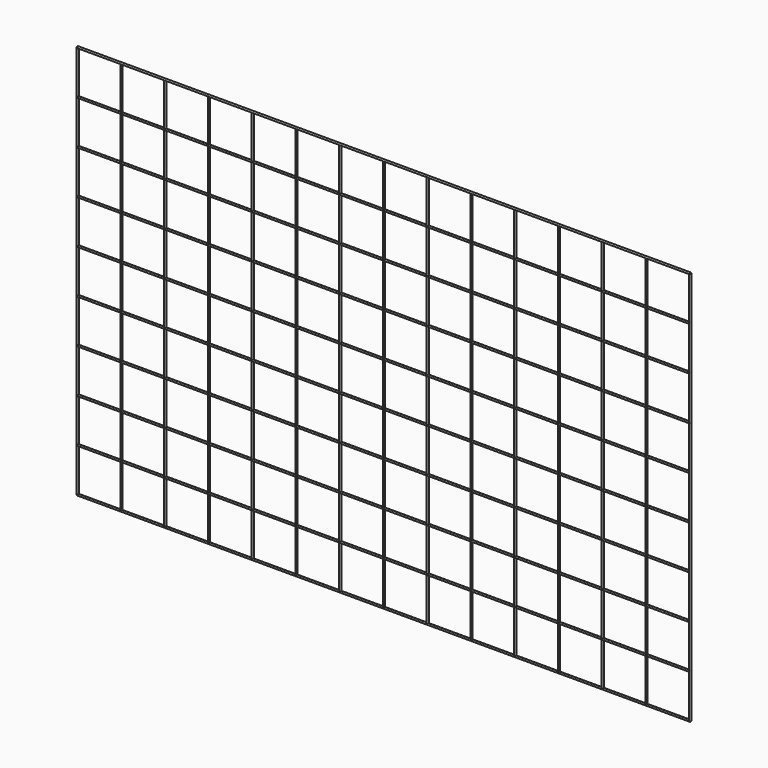
from build123d import *

# Parameters (mm, degrees)
F1_DEPTH = 2800
F2_R     = 4
F3_DEPTH = 1800


with BuildPart() as f1:
    # F0 (on Right) → F1 (new body)
    with BuildSketch(Plane.YZ):
        with BuildLine():
            ThreePointArc((4, -1800), (2.8284271247, -1797.1715728753), (0, -1796))
            ThreePointArc((0, -1796), (-2.8284271247, -1802.8284271247), (4, -1800))
        make_face()
    extrude(amount=F1_DEPTH)


with BuildPart() as f1b:
    # F0 (on Right) → F1, piece 2 (new body)
    with BuildSketch(Plane.YZ):
        with BuildLine():
            ThreePointArc((4, -1600), (2.8284271247, -1597.1715728753), (0, -1596))
            Line((0, -1596), (0, -1600))
            Line((0, -1600), (0, -1604))
            ThreePointArc((0, -1604), (2.8284271247, -1602.8284271247), (4, -1600))
        make_face()
        with BuildLine():
            Line((0, -1600), (0, -1596))
            ThreePointArc((0, -1596), (-4, -1600), (0, -1604))
            Line((0, -1604), (0, -1600))
        make_face()
    extrude(amount=F1_DEPTH)


with BuildPart() as f1c:
    # F0 (on Right) → F1, piece 3 (new body)
    with BuildSketch(Plane.YZ):
        with BuildLine():
            ThreePointArc((4, -1400), (2.8284271247, -1397.1715728753), (0, -1396))
            Line((0, -1396), (0, -1400))
            Line((0, -1400), (0, -1404))
            ThreePointArc((0, -1404), (2.8284271247, -1402.8284271247), (4, -1400))
        make_face()
        with BuildLine():
            Line((0, -1400), (0, -1396))
            ThreePointArc((0, -1396), (-4, -1400), (0, -1404))
            Line((0, -1404), (0, -1400))
        make_face()
    extrude(amount=F1_DEPTH)


with BuildPart() as f1d:
    # F0 (on Right) → F1, piece 4 (new body)
    with BuildSketch(Plane.YZ):
        with BuildLine():
            ThreePointArc((4, -1200), (2.8284271247, -1197.1715728753), (0, -1196))
            Line((0, -1196), (0, -1200))
            Line((0, -1200), (0, -1204))
            ThreePointArc((0, -1204), (2.8284271247, -1202.8284271247), (4, -1200))
        make_face()
        with BuildLine():
            Line((0, -1200), (0, -1196))
            ThreePointArc((0, -1196), (-4, -1200), (0, -1204))
            Line((0, -1204), (0, -1200))
        make_face()
    extrude(amount=F1_DEPTH)


with BuildPart() as f1e:
    # F0 (on Right) → F1, piece 5 (new body)
    with BuildSketch(Plane.YZ):
        with BuildLine():
            ThreePointArc((4, -1000), (2.8284271247, -997.1715728753), (0, -996))
            Line((0, -996), (0, -1000))
            Line((0, -1000), (0, -1004))
            ThreePointArc((0, -1004), (2.8284271247, -1002.8284271247), (4, -1000))
        make_face()
        with BuildLine():
            Line((0, -1000), (0, -996))
            ThreePointArc((0, -996), (-4, -1000), (0, -1004))
            Line((0, -1004), (0, -1000))
        make_face()
    extrude(amount=F1_DEPTH)


with BuildPart() as f1f:
    # F0 (on Right) → F1, piece 6 (new body)
    with BuildSketch(Plane.YZ):
        with BuildLine():
            ThreePointArc((4, -800), (2.8284271247, -797.1715728753), (0, -796))
            Line((0, -796), (0, -800))
            Line((0, -800), (0, -804))
            ThreePointArc((0, -804), (2.8284271247, -802.8284271247), (4, -800))
        make_face()
        with BuildLine():
            Line((0, -800), (0, -796))
            ThreePointArc((0, -796), (-4, -800), (0, -804))
            Line((0, -804), (0, -800))
        make_face()
    extrude(amount=F1_DEPTH)


with BuildPart() as f1g:
    # F0 (on Right) → F1, piece 7 (new body)
    with BuildSketch(Plane.YZ):
        with BuildLine():
            ThreePointArc((4, -600), (2.8284271247, -597.1715728753), (0, -596))
            Line((0, -596), (0, -600))
            Line((0, -600), (0, -604))
            ThreePointArc((0, -604), (2.8284271247, -602.8284271247), (4, -600))
        make_face()
        with BuildLine():
            Line((0, -600), (0, -596))
            ThreePointArc((0, -596), (-4, -600), (0, -604))
            Line((0, -604), (0, -600))
        make_face()
    extrude(amount=F1_DEPTH)


with BuildPart() as f1h:
    # F0 (on Right) → F1, piece 8 (new body)
    with BuildSketch(Plane.YZ):
        with BuildLine():
            ThreePointArc((4, -400), (2.8284271247, -397.1715728753), (0, -396))
            Line((0, -396), (0, -400))
            Line((0, -400), (0, -404))
            ThreePointArc((0, -404), (2.8284271247, -402.8284271247), (4, -400))
        make_face()
        with BuildLine():
            Line((0, -400), (0, -396))
            ThreePointArc((0, -396), (-4, -400), (0, -404))
            Line((0, -404), (0, -400))
        make_face()
    extrude(amount=F1_DEPTH)


with BuildPart() as f1i:
    # F0 (on Right) → F1, piece 9 (new body)
    with BuildSketch(Plane.YZ):
        with BuildLine():
            ThreePointArc((4, -200), (2.8284271247, -197.1715728753), (0, -196))
            Line((0, -196), (0, -200))
            Line((0, -200), (0, -204))
            ThreePointArc((0, -204), (2.8284271247, -202.8284271247), (4, -200))
        make_face()
        with BuildLine():
            Line((0, -200), (0, -196))
            ThreePointArc((0, -196), (-4, -200), (0, -204))
            Line((0, -204), (0, -200))
        make_face()
    extrude(amount=F1_DEPTH)


with BuildPart() as f1j:
    # F0 (on Right) → F1, piece 10 (new body)
    with BuildSketch(Plane.YZ):
        with BuildLine():
            ThreePointArc((4, 0), (-2.8284271247, 2.8284271247), (0, -4))
            ThreePointArc((0, -4), (2.8284271247, -2.8284271247), (4, 0))
        make_face()
    extrude(amount=F1_DEPTH)

    # F2 (on Top) → F3 (join)
    with BuildSketch(Plane.XY):
        with BuildLine():
            ThreePointArc((2804, 0), (2800, 4), (2796, 0))
            ThreePointArc((2796, 0), (2800, -4), (2804, 0))
        make_face()
        with BuildLine():
            ThreePointArc((2604, 0), (2600, 4), (2596, 0))
            Line((2596, 0), (2600, 0))
            Line((2600, 0), (2604, 0))
        make_face()
        with BuildLine():
            Line((2600, 0), (2596, 0))
            ThreePointArc((2596, 0), (2600, -4), (2604, 0))
            Line((2604, 0), (2600, 0))
        make_face()
        with BuildLine():
            ThreePointArc((2404, 0), (2400, 4), (2396, 0))
            Line((2396, 0), (2400, 0))
            Line((2400, 0), (2404, 0))
        make_face()
        with BuildLine():
            Line((2400, 0), (2396, 0))
            ThreePointArc((2396, 0), (2400, -4), (2404, 0))
            Line((2404, 0), (2400, 0))
        make_face()
        with BuildLine():
            ThreePointArc((2204, 0), (2200, 4), (2196, 0))
            Line((2196, 0), (2200, 0))
            Line((2200, 0), (2204, 0))
        make_face()
        with BuildLine():
            Line((2200, 0), (2196, 0))
            ThreePointArc((2196, 0), (2200, -4), (2204, 0))
            Line((2204, 0), (2200, 0))
        make_face()
        with BuildLine():
            ThreePointArc((2004, 0), (2000, 4), (1996, 0))
            Line((1996, 0), (2000, 0))
            Line((2000, 0), (2004, 0))
        make_face()
        with BuildLine():
            Line((2000, 0), (1996, 0))
            ThreePointArc((1996, 0), (2000, -4), (2004, 0))
            Line((2004, 0), (2000, 0))
        make_face()
        with BuildLine():
            ThreePointArc((1804, 0), (1800, 4), (1796, 0))
            Line((1796, 0), (1800, 0))
            Line((1800, 0), (1804, 0))
        make_face()
        with BuildLine():
            Line((1800, 0), (1796, 0))
            ThreePointArc((1796, 0), (1800, -4), (1804, 0))
            Line((1804, 0), (1800, 0))
        make_face()
        with BuildLine():
            ThreePointArc((1604, 0), (1600, 4), (1596, 0))
            Line((1596, 0), (1600, 0))
            Line((1600, 0), (1604, 0))
        make_face()
        with BuildLine():
            Line((1600, 0), (1596, 0))
            ThreePointArc((1596, 0), (1600, -4), (1604, 0))
            Line((1604, 0), (1600, 0))
        make_face()
        with BuildLine():
            ThreePointArc((1404, 0), (1400, 4), (1396, 0))
            Line((1396, 0), (1400, 0))
            Line((1400, 0), (1404, 0))
        make_face()
        with BuildLine():
            Line((1400, 0), (1396, 0))
            ThreePointArc((1396, 0), (1400, -4), (1404, 0))
            Line((1404, 0), (1400, 0))
        make_face()
        with BuildLine():
            ThreePointArc((1204, 0), (1200, 4), (1196, 0))
            Line((1196, 0), (1200, 0))
            Line((1200, 0), (1204, 0))
        make_face()
        with BuildLine():
            Line((1200, 0), (1196, 0))
            ThreePointArc((1196, 0), (1200, -4), (1204, 0))
            Line((1204, 0), (1200, 0))
        make_face()
        with BuildLine():
            ThreePointArc((1004, 0), (1000, 4), (996, 0))
            Line((996, 0), (1000, 0))
            Line((1000, 0), (1004, 0))
        make_face()
        with BuildLine():
            Line((1000, 0), (996, 0))
            ThreePointArc((996, 0), (1000, -4), (1004, 0))
            Line((1004, 0), (1000, 0))
        make_face()
        with BuildLine():
            ThreePointArc((804, 0), (800, 4), (796, 0))
            Line((796, 0), (800, 0))
            Line((800, 0), (804, 0))
        make_face()
        with BuildLine():
            Line((800, 0), (796, 0))
            ThreePointArc((796, 0), (800, -4), (804, 0))
            Line((804, 0), (800, 0))
        make_face()
        with BuildLine():
            ThreePointArc((604, 0), (600, 4), (596, 0))
            Line((596, 0), (600, 0))
            Line((600, 0), (604, 0))
        make_face()
        with BuildLine():
            Line((600, 0), (596, 0))
            ThreePointArc((596, 0), (600, -4), (604, 0))
            Line((604, 0), (600, 0))
        make_face()
        with BuildLine():
            ThreePointArc((404, 0), (400, 4), (396, 0))
            Line((396, 0), (400, 0))
            Line((400, 0), (404, 0))
        make_face()
        with BuildLine():
            Line((400, 0), (396, 0))
            ThreePointArc((396, 0), (400, -4), (404, 0))
            Line((404, 0), (400, 0))
        make_face()
        with BuildLine():
            ThreePointArc((204, 0), (200, 4), (196, 0))
            Line((196, 0), (200, 0))
            Line((200, 0), (204, 0))
        make_face()
        with BuildLine():
            Line((200, 0), (196, 0))
            ThreePointArc((196, 0), (200, -4), (204, 0))
            Line((204, 0), (200, 0))
        make_face()
        Circle(F2_R)
    extrude(amount=-F3_DEPTH)


solid = Compound([f1.part, f1b.part, f1c.part, f1d.part, f1e.part, f1f.part, f1g.part, f1h.part, f1i.part, f1j.part])
